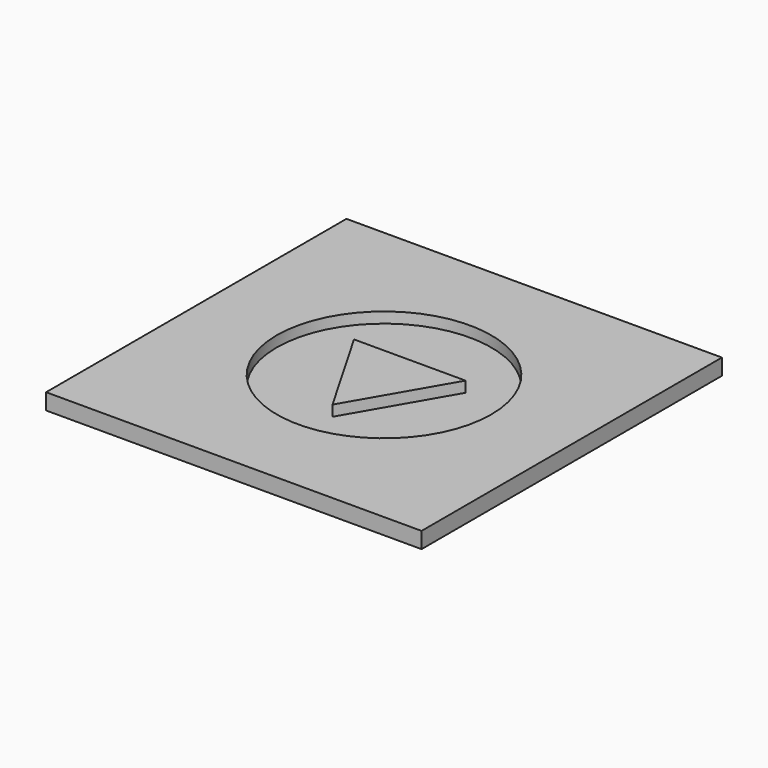
from build123d import *

# Parameters (mm, degrees)
F0_W     = 70
F0_H     = 70
F0_R     = 20
F1_DEPTH = 2
F2_DEPTH = 1


# Not quite as in the source:
# - a feature names something its author has since deleted; it is built from what else it names


with BuildPart() as f1:
    # F0 (on Top) → F1 (new body)
    with BuildSketch(Plane.XY):
        Rectangle(F0_W, F0_H)
        Circle(F0_R, mode=Mode.SUBTRACT)
    extrude(amount=F1_DEPTH)



with BuildPart() as f1b:
    # F0 (on Top) → F1, piece 2 (new body)
    with BuildSketch(Plane.XY):
        Polygon((10.3923048454, 6), (-10.3923048454, 6), (0, -12), align=None)
    extrude(amount=F1_DEPTH)


with BuildPart() as f1_1:
    add(f1.part)

    add(f1b.part)  # F2 merges F1b
    # F0 (on Top) → F2 (join)
    with BuildSketch(Plane.XY):
        Rectangle(F0_W, F0_H)
        Circle(F0_R, mode=Mode.SUBTRACT)
        Circle(F0_R)
        Polygon((0, -12), (-10.3923048454, 6), (10.3923048454, 6), align=None, mode=Mode.SUBTRACT)
        Polygon((10.3923048454, 6), (-10.3923048454, 6), (0, -12), align=None)
    extrude(amount=-F2_DEPTH)


solid = f1_1.part
